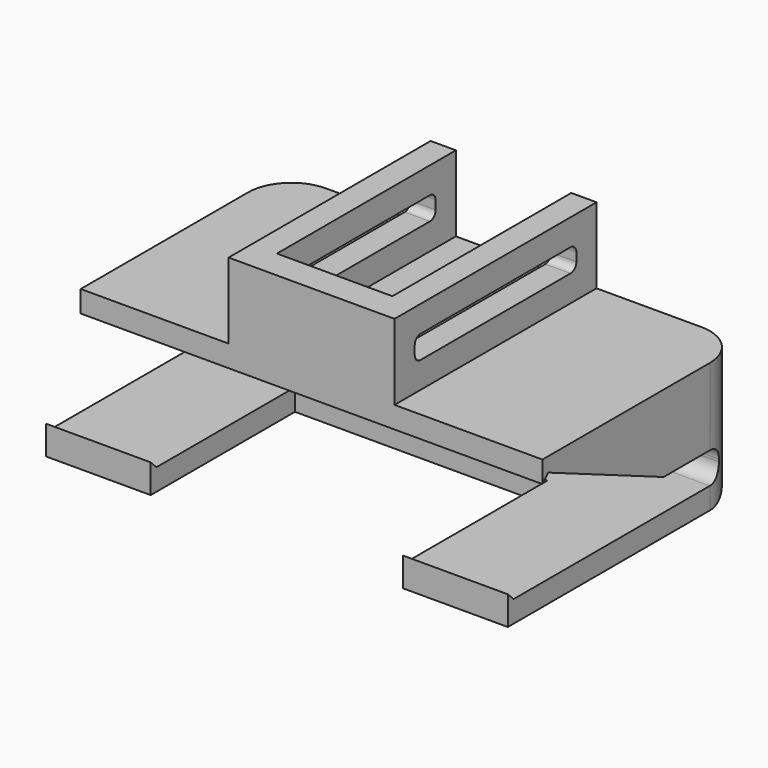
from build123d import *

# Parameters (mm, degrees)
F1_DEPTH     = 32
F3_DEPTH     = 64
F4_W         = 3.5
F4_H         = 35
F5_DEPTH     = 10.5
F7_DEPTH     = 3.5
F8_W         = 16
F8_H         = 4
F9_DEPTH     = 10.5
F10_T1_DEPTH = 48
F10_T3_DEPTH = 94
F11_W        = 35
F11_H        = 25
F12_DEPTH    = 4.001
F13_R        = 2


# Not quite as in the source:
# - a fillet or chamfer that OpenCascade refuses, or shapes differently, is made with other operations: its cross-section is extruded or revolved along the edge and cut away or added
# - a pattern or mirror of a feature is missing from the dataset's text; its kind, count and spacing are read off the source's solid


with BuildPart() as f1:
    # F0 (on Right) → F1 (new body, symmetric)
    with BuildSketch(Plane.YZ):
        Polygon((13.5, -6), (-22.5, -6), (-23.5, -5), (-23.5, -9), (17.5, -9), (17.5, 9), (-17.5, 9), (-17.5, 6), (-16.5, 7), align=None)
    extrude(amount=F1_DEPTH, both=True)

    # F2 (on face) → F3 (cut, through all)
    with BuildSketch(Plane.YZ.offset(32)):
        with BuildLine():
            Line((3.5, -1.6666666667), (13.5, -6))
            Line((13.5, -6), (13.5, -3.6666666667))
            ThreePointArc((13.5, -3.6666666667), (12.9142135624, -2.2524531043), (11.5, -1.6666666667))
            Line((11.5, -1.6666666667), (3.5, -1.6666666667))
        make_face()
    extrude(amount=-F3_DEPTH, mode=Mode.SUBTRACT)

    # F4 (on face) → F5 (join)
    with BuildSketch(Plane.XY.offset(9)):
        with Locations((-9.75, 0)):
            Rectangle(F4_W, F4_H)
    f5 = extrude(amount=F5_DEPTH)

    # F5_copies: F5 across plane
    add(f5.mirror(Plane(origin=(0, 0, 0), x_dir=(0, 0, 1), z_dir=(1, 0, 0))))

    # F6 (on face) → F7 (cut, through all)
    with BuildSketch(Plane(origin=(-11.5, 0, 0), x_dir=(0, -1, 0), z_dir=(-1, 0, 0))):
        with BuildLine():
            Line((13, 15.85), (-13, 15.85))
            ThreePointArc((-13, 15.85), (-13.7071067812, 15.5571067812), (-14, 14.85))
            Line((-14, 14.85), (-14, 13.65))
            ThreePointArc((-14, 13.65), (-13.7071067812, 12.9428932188), (-13, 12.65))
            Line((-13, 12.65), (13, 12.65))
            ThreePointArc((13, 12.65), (13.7071067812, 12.9428932188), (14, 13.65))
            Line((14, 13.65), (14, 14.85))
            ThreePointArc((14, 14.85), (13.7071067812, 15.5571067812), (13, 15.85))
        make_face()
    f7 = extrude(amount=-F7_DEPTH, mode=Mode.SUBTRACT)

    # F7_copies: F7 across plane
    add(f7.mirror(Plane(origin=(0, 0, 0), x_dir=(0, 0, 1), z_dir=(1, 0, 0))), mode=Mode.SUBTRACT)

    # F8 (on face) → F9 (join, through all)
    with BuildSketch(Plane.XY.offset(9)):
        with Locations((0, -15.5)):
            Rectangle(F8_W, F8_H)
    extrude(amount=F9_DEPTH)

    # F10: fillet of radius 6 on 3 edges, made by hand

    # F10_s2 → F10_t1 (cut)
    with BuildSketch(Plane.XY.offset(-24)):
        with BuildLine():
            ThreePointArc((26, 17.5), (30.2426406871, 15.7426406871), (32, 11.5))
            Line((32, 11.5), (32, 17.5))
            Line((32, 17.5), (26, 17.5))
        make_face()
        with BuildLine():
            ThreePointArc((-26, 17.5), (-30.2426406871, 15.7426406871), (-32, 11.5))
            Line((-32, 11.5), (-32, 17.5))
            Line((-32, 17.5), (-26, 17.5))
        make_face()
    extrude(amount=F10_T1_DEPTH, mode=Mode.SUBTRACT)

    # F10_s4 → F10_t3 (cut)
    with BuildSketch(Plane.YZ.offset(-47)):
        with BuildLine():
            ThreePointArc((17.5, -3), (15.7426406871, -7.2426406871), (11.5, -9))
            Line((11.5, -9), (17.5, -9))
            Line((17.5, -9), (17.5, -3))
        make_face()
    extrude(amount=F10_T3_DEPTH, mode=Mode.SUBTRACT)

    # F11 (on face) → F12 (cut, through all)
    with BuildSketch(Plane(origin=(0, 0, -9), x_dir=(1, 0, 0), z_dir=(0, 0, -1))):
        with Locations((0, 11)):
            Rectangle(F11_W, F11_H)
    extrude(amount=-F12_DEPTH, mode=Mode.SUBTRACT)

    # F13
    f13_edges = [f1.edges().sort_by_distance(p)[0] for p in [
        (0, 13.5, -6),
    ]]
    fillet(f13_edges, radius=F13_R)


solid = f1.part
